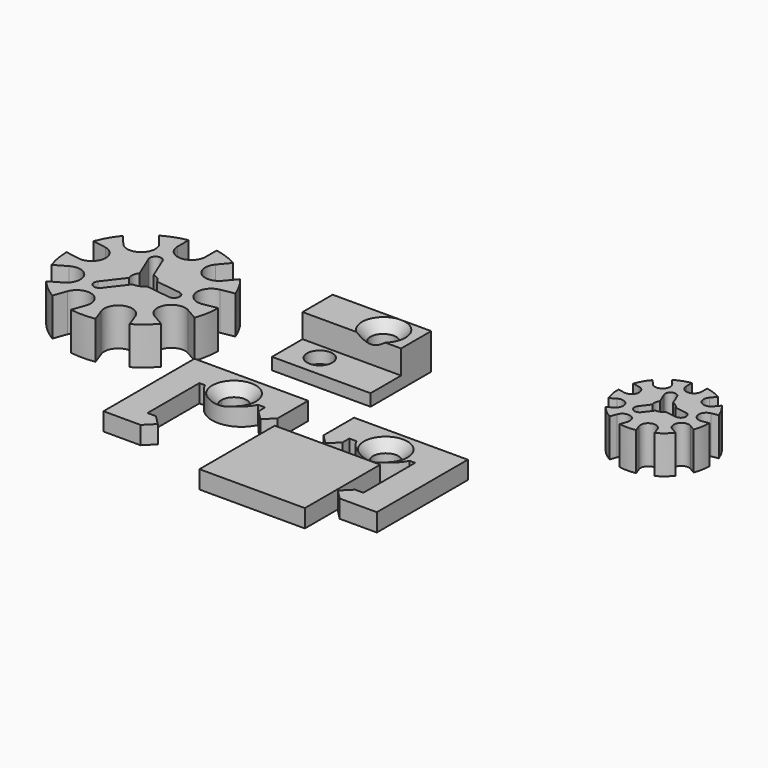
from build123d import *

# Parameters (mm, degrees)
F0_W      = 16.51
F0_H      = 12.7
F0_R      = 2.125
F1_DEPTH  = 2
F2_W      = 16.51
F2_H      = 6.3
F2_R      = 2.125
F3_DEPTH  = 4
F5_DEPTH  = 3
F14_DEPTH = 6.35


# Not quite as in the source:
# - a feature names something its author has since deleted; it is built from what else it names


with BuildPart() as f1:
    # F0 (on Top) → F1 (new body)
    with BuildSketch(Plane.XY):
        with Locations((-8.255, 6.35)):
            Rectangle(F0_W, F0_H)
        with Locations((-11.43, 3.65)):
            Circle(F0_R, mode=Mode.SUBTRACT)
        with Locations((-5.08, 9.05)):
            Circle(F0_R, mode=Mode.SUBTRACT)
    extrude(amount=F1_DEPTH)

    # F2 (on face) → F3 (join)
    with BuildSketch(Plane.XY.offset(2)):
        with Locations((-8.255, 9.55)):
            Rectangle(F2_W, F2_H)
        with Locations((-5.08, 9.05)):
            Circle(F2_R, mode=Mode.SUBTRACT)
    extrude(amount=F3_DEPTH)

    # F11 (on offset) → F12 (revolve, cut)
    with BuildSketch(Plane.XZ.offset(-9.0924)):
        Polygon((-5.08, 4.095), (-5.08, 6), (-8.7002697044, 6), (-6.985, 4.095), align=None)
    revolve(axis=Axis((-5.08, 9.0924, 4.5872520752), (0, 0, -1)), mode=Mode.SUBTRACT)


with BuildPart() as f5:
    # F4 (on Top) → F5 (new body)
    with BuildSketch(Plane.XY):
        with BuildLine():
            ThreePointArc((14.7509726961, -13.256), (12.7, -14.825), (10.6490273039, -13.256))
            Line((10.6490273039, -13.256), (8.255, -13.256))
            ThreePointArc((8.255, -13.256), (12.7, -16.0680154632), (17.145, -13.256))
            Line((17.145, -13.256), (14.7509726961, -13.256))
        make_face()
        with BuildLine():
            ThreePointArc((10.6490273039, -13.256), (12.4195467767, -10.5935881244), (14.825, -12.7))
            ThreePointArc((14.825, -12.7), (14.8064118756, -12.9804532233), (14.7509726961, -13.256))
            Line((14.7509726961, -13.256), (17.145, -13.256))
            Line((17.145, -13.256), (18.079, -13.256))
            Line((18.079, -13.256), (18.079, -24.1020883642))
            Line((18.079, -24.1020883642), (16.6804558179, -24.1020883642))
            Line((16.6804558179, -24.1020883642), (15.079, -25.7035441821))
            Line((15.079, -25.7035441821), (16.6804558179, -27.305))
            Line((16.6804558179, -27.305), (22.8972320884, -27.305))
            Line((22.8972320884, -27.305), (22.8972320884, -8.255))
            Line((22.8972320884, -8.255), (3.8472320884, -8.255))
            Line((3.8472320884, -8.255), (3.8472320884, -14.6545441821))
            Line((3.8472320884, -14.6545441821), (5.4486879063, -16.256))
            Line((5.4486879063, -16.256), (7.0501437242, -14.6545441821))
            Line((7.0501437242, -14.6545441821), (7.0501437242, -13.256))
            Line((7.0501437242, -13.256), (8.255, -13.256))
            Line((8.255, -13.256), (10.6490273039, -13.256))
        make_face()
    extrude(amount=F5_DEPTH)

    # F7 (on offset) → F8 (revolve, cut)
    with BuildSketch(Plane(origin=(0, -12.7, 0), x_dir=(-1, 0, 0), z_dir=(0, 1, 0))):
        Polygon((-12.7, 1.095), (-12.7, 3), (-16.3506108865, 3), (-14.605, 1.095), align=None)
    revolve(axis=Axis((12.7, -12.7, 2.0475), (0, 0, 1)), mode=Mode.SUBTRACT)


with BuildPart() as f5b:
    # F4 (on Top) → F5, piece 2 (new body)
    with BuildSketch(Plane.XY):
        Polygon((14.825, -16.51), (3.8472320884, -16.51), (-2.8377089754, -16.51), (-2.8377089754, -32.2849750519), (14.825, -32.2849750519), align=None)
    extrude(amount=F5_DEPTH)


with BuildPart() as f9_1:
    # F9: instance of F5
    add(f5.part.mirror(Plane.YZ))


with BuildPart() as f14:
    # F13 (on Top) → F14 (new body)
    with BuildSketch(Plane.XY):
        with BuildLine():
            Line((-28.5023396228, 4.0780713008), (-26.2168182614, 4.4810703818))
            ThreePointArc((-26.2168182614, 4.4810703818), (-27.1014773719, 6.35), (-28.2776883439, 8.0506020725))
            Line((-28.2776883439, 8.0506020725), (-29.7694564665, 6.2727820531))
            ThreePointArc((-29.7694564665, 6.2727820531), (-33.0795073745, 5.983190123), (-33.3690993047, 9.293241031))
            Line((-33.3690993047, 9.293241031), (-31.8773311821, 11.0710610505))
            ThreePointArc((-31.8773311821, 11.0710610505), (-33.7563441798, 11.934096284), (-35.7505, 12.4807792125))
            Line((-35.7505, 12.4807792125), (-35.7505, 10.16))
            ThreePointArc((-35.7505, 10.16), (-38.1, 7.8105), (-40.4495, 10.16))
            Line((-40.4495, 10.16), (-40.4495, 12.4807792125))
            ThreePointArc((-40.4495, 12.4807792125), (-42.4436558202, 11.934096284), (-44.3226688179, 11.0710610505))
            Line((-44.3226688179, 11.0710610505), (-42.8309006953, 9.293241031))
            ThreePointArc((-42.8309006953, 9.293241031), (-43.1204926255, 5.983190123), (-46.4305435335, 6.2727820531))
            Line((-46.4305435335, 6.2727820531), (-47.9223116561, 8.0506020725))
            ThreePointArc((-47.9223116561, 8.0506020725), (-49.0985226281, 6.35), (-49.9831817386, 4.4810703818))
            Line((-49.9831817386, 4.4810703818), (-47.6976603772, 4.0780713008))
            ThreePointArc((-47.6976603772, 4.0780713008), (-45.7918409549, 1.3562790917), (-48.513633164, -0.5495403306))
            Line((-48.513633164, -0.5495403306), (-50.7991545255, -0.1465412496))
            ThreePointArc((-50.7991545255, -0.1465412496), (-50.6070584633, -2.2053318564), (-50.083421857, -4.20566292))
            Line((-50.083421857, -4.20566292), (-48.0735681024, -3.0452733138))
            ThreePointArc((-48.0735681024, -3.0452733138), (-44.8640914163, -3.90525), (-45.7240681024, -7.1147266862))
            Line((-45.7240681024, -7.1147266862), (-47.733921857, -8.2751162924))
            ThreePointArc((-47.733921857, -8.2751162924), (-46.263402643, -9.7287644276), (-44.5764857076, -10.9245198009))
            Line((-44.5764857076, -10.9245198009), (-43.7827324687, -8.7437007004))
            ThreePointArc((-43.7827324687, -8.7437007004), (-40.7713483294, -7.3394692146), (-39.3671168437, -10.3508533539))
            Line((-39.3671168437, -10.3508533539), (-40.1608700825, -12.5316724543))
            ThreePointArc((-40.1608700825, -12.5316724543), (-38.1, -12.7), (-36.0391299175, -12.5316724543))
            Line((-36.0391299175, -12.5316724543), (-36.8328831563, -10.3508533539))
            ThreePointArc((-36.8328831563, -10.3508533539), (-35.4286516706, -7.3394692146), (-32.4172675313, -8.7437007004))
            Line((-32.4172675313, -8.7437007004), (-31.6235142924, -10.9245198009))
            ThreePointArc((-31.6235142924, -10.9245198009), (-29.936597357, -9.7287644276), (-28.466078143, -8.2751162924))
            Line((-28.466078143, -8.2751162924), (-30.4759318976, -7.1147266862))
            ThreePointArc((-30.4759318976, -7.1147266862), (-31.3359085837, -3.90525), (-28.1264318976, -3.0452733138))
            Line((-28.1264318976, -3.0452733138), (-26.116578143, -4.20566292))
            ThreePointArc((-26.116578143, -4.20566292), (-25.5929415367, -2.2053318564), (-25.4008454745, -0.1465412496))
            Line((-25.4008454745, -0.1465412496), (-27.686366836, -0.5495403306))
            ThreePointArc((-27.686366836, -0.5495403306), (-30.4081590451, 1.3562790917), (-28.5023396228, 4.0780713008))
        make_face()
        with BuildLine():
            ThreePointArc((-37.8513476038, 1.8887024609), (-36.9403094777, 1.5113381133), (-36.3400094906, 0.7290119387))
            Line((-36.3400094906, 0.7290119387), (-32.1848640765, 0.1819766671))
            ThreePointArc((-32.1848640765, 0.1819766671), (-31.3648390442, -0.8867007615), (-32.4335164727, -1.7067257939))
            Line((-32.4335164727, -1.7067257939), (-36.5886618867, -1.1596905223))
            ThreePointArc((-36.5886618867, -1.1596905223), (-37.3709880613, -1.7599905094), (-38.3486523962, -1.8887024609))
            Line((-38.3486523962, -1.8887024609), (-40.8999715452, -5.2136463101))
            ThreePointArc((-40.8999715452, -5.2136463101), (-42.2354858629, -5.3894701056), (-42.4113096584, -4.0539557878))
            Line((-42.4113096584, -4.0539557878), (-39.8599905094, -0.7290119387))
            ThreePointArc((-39.8599905094, -0.7290119387), (-39.9887024609, 0.2486523962), (-39.6113381133, 1.1596905223))
            Line((-39.6113381133, 1.1596905223), (-41.2151643783, 5.031669643))
            ThreePointArc((-41.2151643783, 5.031669643), (-40.6996750929, 6.2761708671), (-39.4551738689, 5.7606815817))
            Line((-39.4551738689, 5.7606815817), (-37.8513476038, 1.8887024609))
        make_face(mode=Mode.SUBTRACT)
    extrude(amount=F14_DEPTH)


with BuildPart() as f14b:
    # F13 (on Top) → F14, piece 2 (new body)
    with BuildSketch(Plane.XY):
        with BuildLine():
            ThreePointArc((44.6448019103, 11.8470276537), (45.0024888463, 13.1541121223), (45.1229881739, 14.5038860532))
            ThreePointArc((45.1229881739, 14.5038860532), (45.1229403632, 14.5308792599), (45.1227969316, 14.5578721279))
            Line((45.1227969316, 14.5578721279), (43.9770505912, 14.355846135))
            ThreePointArc((43.9770505912, 14.355846135), (42.5058115592, 15.3860187957), (43.5359842199, 16.8572578277))
            Line((43.5359842199, 16.8572578277), (44.6817305603, 17.0592838205))
            ThreePointArc((44.6817305603, 17.0592838205), (44.1021017507, 18.3138860532), (43.3053987504, 19.4431604433))
            Line((43.3053987504, 19.4431604433), (42.5575659382, 18.5519280027))
            ThreePointArc((42.5575659382, 18.5519280027), (40.7683492311, 18.3953918242), (40.6118130526, 20.1846085313))
            Line((40.6118130526, 20.1846085313), (41.3596458649, 21.0758409719))
            ThreePointArc((41.3596458649, 21.0758409719), (40.109181666, 21.6643438236), (38.7729881739, 22.0173073777))
            Line((38.7729881739, 22.0173073777), (38.7729881739, 20.8538860532))
            ThreePointArc((38.7729881739, 20.8538860532), (37.5029881739, 19.5838860532), (36.2329881739, 20.8538860532))
            Line((36.2329881739, 20.8538860532), (36.2329881739, 22.0173073777))
            ThreePointArc((36.2329881739, 22.0173073777), (34.8967946818, 21.6643438236), (33.6463304829, 21.0758409719))
            Line((33.6463304829, 21.0758409719), (34.3941632951, 20.1846085313))
            ThreePointArc((34.3941632951, 20.1846085313), (34.2376271167, 18.3953918242), (32.4484104096, 18.5519280027))
            Line((32.4484104096, 18.5519280027), (31.7005775974, 19.4431604433))
            ThreePointArc((31.7005775974, 19.4431604433), (30.9038745971, 18.3138860532), (30.3242457875, 17.0592838205))
            Line((30.3242457875, 17.0592838205), (31.4699921279, 16.8572578277))
            ThreePointArc((31.4699921279, 16.8572578277), (32.5001647886, 15.3860187957), (31.0289257566, 14.355846135))
            Line((31.0289257566, 14.355846135), (29.8831794162, 14.5578721279))
            ThreePointArc((29.8831794162, 14.5578721279), (29.9987530959, 13.1806869393), (30.3611744375, 11.8470276537))
            Line((30.3611744375, 11.8470276537), (31.3687268599, 12.428738316))
            ThreePointArc((31.3687268599, 12.428738316), (33.1035791227, 11.9638860532), (32.6387268599, 10.2290337904))
            Line((32.6387268599, 10.2290337904), (31.6311744375, 9.6473231281))
            ThreePointArc((31.6311744375, 9.6473231281), (32.6049465881, 8.6666273966), (33.7398371072, 7.8779450597))
            Line((33.7398371072, 7.8779450597), (34.1377506354, 8.9712034932))
            ThreePointArc((34.1377506354, 8.9712034932), (35.7655258458, 9.7302475396), (36.5245698922, 8.1024723292))
            Line((36.5245698922, 8.1024723292), (36.126656364, 7.0092138956))
            ThreePointArc((36.126656364, 7.0092138956), (37.5029881739, 6.8838860532), (38.8793199838, 7.0092138956))
            Line((38.8793199838, 7.0092138956), (38.4814064556, 8.1024723292))
            ThreePointArc((38.4814064556, 8.1024723292), (39.240450502, 9.7302475396), (40.8682257124, 8.9712034932))
            Line((40.8682257124, 8.9712034932), (41.2661392406, 7.8779450597))
            ThreePointArc((41.2661392406, 7.8779450597), (42.4010297597, 8.6666273966), (43.3748019103, 9.6473231281))
            Line((43.3748019103, 9.6473231281), (42.3672494879, 10.2290337904))
            ThreePointArc((42.3672494879, 10.2290337904), (41.9023972251, 11.9638860532), (43.6372494879, 12.428738316))
            Line((43.6372494879, 12.428738316), (44.6448019103, 11.8470276537))
        make_face()
        with BuildLine():
            ThreePointArc((37.8209995769, 16.0592075625), (38.4693969424, 15.7633344809), (38.9230059803, 15.2136083083))
            Line((38.9230059803, 15.2136083083), (40.8117084412, 14.9649559121))
            ThreePointArc((40.8117084412, 14.9649559121), (41.5770651381, 13.9675236455), (40.5796328715, 13.2021669486))
            Line((40.5796328715, 13.2021669486), (38.6909304106, 13.4508193448))
            ThreePointArc((38.6909304106, 13.4508193448), (38.1104981228, 13.0372272953), (37.4076167732, 12.9192534314))
            Line((37.4076167732, 12.9192534314), (36.247926251, 11.4079153182))
            ThreePointArc((36.247926251, 11.4079153182), (35.0014462211, 11.243813109), (34.8373440119, 12.4902931389))
            Line((34.8373440119, 12.4902931389), (35.9970345342, 14.0016312522))
            ThreePointArc((35.9970345342, 14.0016312522), (35.9290694565, 14.7110963833), (36.1783417681, 15.3787964198))
            Line((36.1783417681, 15.3787964198), (35.4493298295, 17.1387869292))
            ThreePointArc((35.4493298295, 17.1387869292), (35.9304531625, 18.300321405), (37.0919876383, 17.819198072))
            Line((37.0919876383, 17.819198072), (37.8209995769, 16.0592075625))
        make_face(mode=Mode.SUBTRACT)
    extrude(amount=F14_DEPTH)


solid = Compound([f1.part, f5.part, f5b.part, f9_1.part, f14.part, f14b.part])
